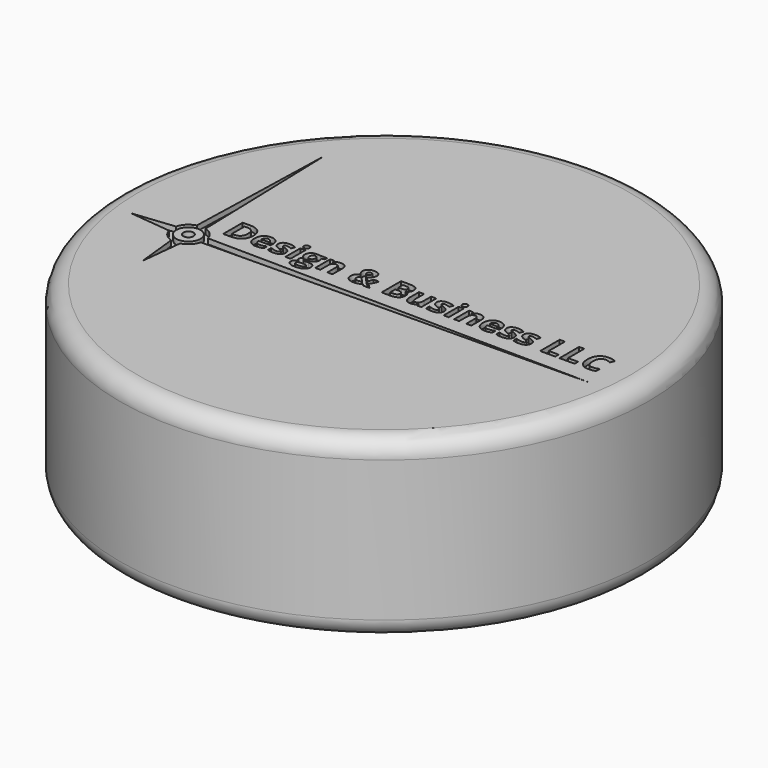
from build123d import *

# Parameters (mm, degrees)
F2_R         = 1.7424001174
F2_TEXT_SIZE = 4.9388888889
F2_R_2       = 0.7280940567
F3_DEPTH     = 0.762


# Not quite as in the source:
# - Text() gives the source's letters only with a copy of the font that has no kerning and outlines rounded to 1/6400 em; it was checked with that copy


with BuildPart() as f1:
    # F0 (on Front) → F1 (revolve)
    with BuildSketch(Plane.XZ):
        with BuildLine():
            Line((0, 25.4), (0, 0))
            Line((0, 0), (35.56, 0))
            ThreePointArc((35.56, 0), (37.3560512242, 0.7439487758), (38.1, 2.54))
            Line((38.1, 2.54), (38.1, 22.86))
            ThreePointArc((38.1, 22.86), (37.3560512242, 24.6560512242), (35.56, 25.4))
            Line((35.56, 25.4), (0, 25.4))
        make_face()
    revolve(axis=Axis((0, 0, 12.7), (0, 0, -1)))

    # F2 (on face) → F3 (cut)
    with BuildSketch(Plane.XY.offset(25.4)):
        with BuildLine():
            ThreePointArc((-22.4558351872, -4.953), (-22.3915115275, -4.6383915157), (-22.3699405228, -4.318))
            ThreePointArc((-22.3699405228, -4.318), (-22.3915115275, -3.9976084843), (-22.4558351872, -3.683))
            ThreePointArc((-22.4558351872, -3.683), (-23.0700003221, -2.6279061381), (-24.125094184, -2.0137410032))
            ThreePointArc((-24.125094184, -2.0137410032), (-24.760094184, -1.9278463388), (-25.395094184, -2.0137410032))
            ThreePointArc((-25.395094184, -2.0137410032), (-26.450188046, -2.6279061381), (-27.0643531808, -3.683))
            ThreePointArc((-27.0643531808, -3.683), (-27.1502478453, -4.318), (-27.0643531808, -4.953))
            ThreePointArc((-27.0643531808, -4.953), (-26.450188046, -6.0080938619), (-25.395094184, -6.6222589968))
            ThreePointArc((-25.395094184, -6.6222589968), (-24.760094184, -6.7081536612), (-24.125094184, -6.6222589968))
            ThreePointArc((-24.125094184, -6.6222589968), (-23.0700003221, -6.0080938619), (-22.4558351872, -4.953))
        make_face()
        with Locations((-24.760094184, -4.318)):
            Circle(F2_R, mode=Mode.SUBTRACT)
        with BuildLine():
            ThreePointArc((-22.4558351872, -3.683), (-22.3915115275, -3.9976084843), (-22.3699405228, -4.318))
            ThreePointArc((-22.3699405228, -4.318), (-22.3915115275, -4.6383915157), (-22.4558351872, -4.953))
            Line((-22.4558351872, -4.953), (33.1704208934, -4.318))
            Line((33.1704208934, -4.318), (-22.4558351872, -3.683))
        make_face()
        with BuildLine():
            ThreePointArc((-25.395094184, -2.0137410032), (-24.760094184, -1.9278463388), (-24.125094184, -2.0137410032))
            Line((-24.125094184, -2.0137410032), (-24.760094184, 19.9372273596))
            Line((-24.760094184, 19.9372273596), (-25.395094184, -2.0137410032))
        make_face()
        with BuildLine():
            Line((-24.760094184, -12.573), (-24.125094184, -6.6222589968))
            ThreePointArc((-24.125094184, -6.6222589968), (-24.760094184, -6.7081536612), (-25.395094184, -6.6222589968))
            Line((-25.395094184, -6.6222589968), (-24.760094184, -12.573))
        make_face()
        with BuildLine():
            ThreePointArc((-27.0643531808, -4.953), (-27.1502478453, -4.318), (-27.0643531808, -3.683))
            Line((-27.0643531808, -3.683), (-33.015094184, -4.318))
            Line((-33.015094184, -4.318), (-27.0643531808, -4.953))
        make_face()
        with Locations((-22.220094184, -1.778)):
            Text('Design & Business LLC', F2_TEXT_SIZE, font='Open Sans', font_style=FontStyle.BOLD, text_align=(TextAlign.LEFT, TextAlign.BOTTOM))
        with Locations((-24.760094184, -4.318)):
            Circle(F2_R_2)
    extrude(amount=-F3_DEPTH, mode=Mode.SUBTRACT)


solid = f1.part
